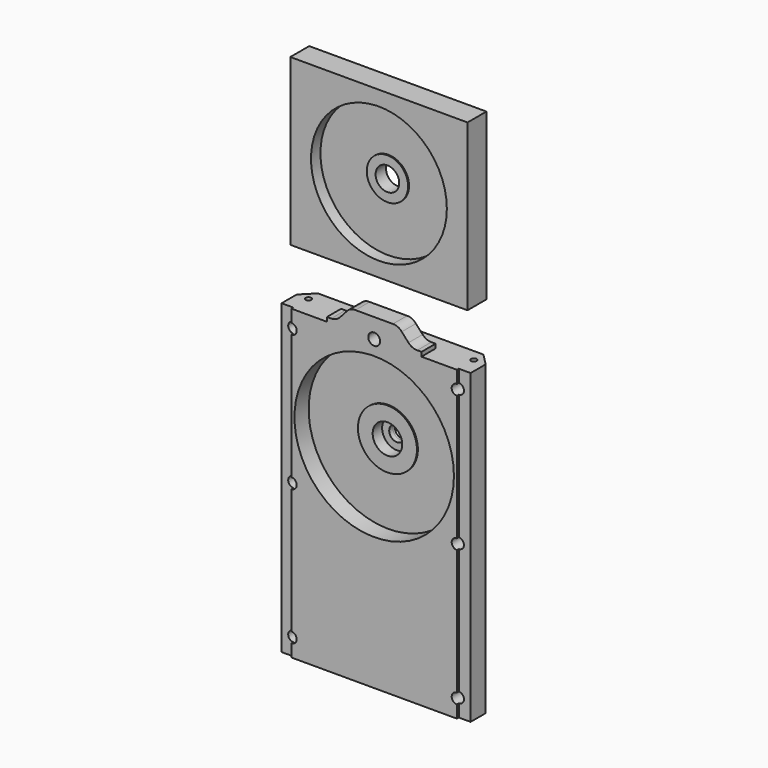
from build123d import *
from build123d import SkipClean  # not in build123d's __all__

# Parameters (mm, degrees)
F0_R            = 3.25
F1_DEPTH        = 6.5
F2_R            = 33.75
F3_DEPTH        = 7.5
F4_R            = 12.5
F4_R_2          = 3.25
F5_DEPTH        = 0.5
F6_R            = 8.25
F6_R_2          = 3.25
F7_DEPTH        = 1
F9_DEPTH        = 50
F10_DEPTH       = 120
F12_D           = 4.4
F12_CBORE_D     = 8.25
F12_CBORE_DEPTH = 4
F13_T1_DEPTH    = 155.7168298797
F14_R           = 2.5
F15_DEPTH       = 15.001
F16_R           = 4.8
F17_DEPTH       = 5
F18_R           = 3.3
F19_DEPTH       = 2.5
F20_R           = 4.8
F21_DEPTH       = 0.1
F23_DEPTH       = 1
F24_R           = 6.25
F25_DEPTH       = 5
F27_D           = 2.4
F27_DEPTH       = 2.5
F27_TIP         = 0.7210327428
F28_W           = 75
F28_H           = 70
F28_R           = 5
F29_DEPTH       = 5
F30_W           = 75
F30_H           = 70
F30_R           = 28.75
F31_DEPTH       = 5
F32_R           = 8.75
F32_R_2         = 5
F33_DEPTH       = 0.5


# Not quite as in the source:
# - a fillet or chamfer that OpenCascade refuses, or shapes differently, is made with other operations: its cross-section is extruded or revolved along the edge and cut away or added
# - after a boolean that leaves OpenCascade's solid faulty, fix() repairs it
# - a feature names something its author has since deleted; it is built from what else it names


with BuildPart() as f1:
    # F0 (on Front) → F1 (new body)
    with BuildSketch(Plane.XZ):
        Polygon((40, -40), (40, -23.2305045641), (40, 0.7694954359), (40, 40), (19.3889045436, 40), (-20.6110954564, 40), (-40, 40), (-40, 0.7694954359), (-40, -23.2305045641), (-40, -40), align=None)
        Circle(F0_R, mode=Mode.SUBTRACT)
    extrude(amount=-F1_DEPTH)

    # F2 (on Front) → F3 (join)
    with BuildSketch(Plane.XZ):
        with BuildLine():
            Line((-40, 40), (-40, -40))
            Line((-40, -40), (40, -40))
            Line((40, -40), (40, 40))
            Line((40, 40), (20, 40))
            Line((20, 40), (20, 41.789))
            Line((20, 41.789), (18.202, 41.789))
            ThreePointArc((18.202, 41.789), (16.1810670348, 42.2156172312), (14.505, 43.4226680199))
            Line((14.505, 43.4226680199), (11.656, 46.56))
            ThreePointArc((11.656, 46.56), (9.9989699318, 47.8636778232), (7.93, 48.2694954359))
            Line((7.93, 48.2694954359), (-7.93, 48.2694954359))
            ThreePointArc((-7.93, 48.2694954359), (-9.9989699318, 47.8636778232), (-11.656, 46.56))
            Line((-11.656, 46.56), (-14.505, 43.4226680199))
            ThreePointArc((-14.505, 43.4226680199), (-16.1810670348, 42.2156172312), (-18.202, 41.789))
            Line((-18.202, 41.789), (-20, 41.789))
            Line((-20, 41.789), (-20, 40))
            Line((-20, 40), (-40, 40))
        make_face()
        Circle(F2_R, mode=Mode.SUBTRACT)
    extrude(amount=F3_DEPTH)

    # F4 (on face) → F5 (join)
    with BuildSketch(Plane.XZ):
        Circle(F4_R)
        Circle(F4_R_2, mode=Mode.SUBTRACT)
    extrude(amount=F5_DEPTH)

    # F6 (on face) → F7 (join)
    with BuildSketch(Plane(origin=(0, 6.5, 0), x_dir=(-1, 0, 0), z_dir=(0, 1, 0))):
        Circle(F6_R)
        Circle(F6_R_2, mode=Mode.SUBTRACT)
    with SkipClean():  # cleaning this boolean's faces spoils the solid; the shape is the same uncleaned
        extrude(amount=F7_DEPTH)

    # F8 (on face) → F9 (join)
    with BuildSketch(Plane(origin=(0, 0, -40), x_dir=(1, 0, 0), z_dir=(0, 0, -1))):
        Polygon((27.5, -6.5), (40, -6.5), (40, 6.5), (35, 6.5), (35, 7.5), (-35, 7.5), (-35, 6.5), (-40, 6.5), (-40, -6.5), (-27.5, -6.5), (-27.5, 2.5), (27.5, 2.5), align=None)
    extrude(amount=F9_DEPTH)

    add(f1.part.fix(), mode=Mode.REPLACE)

    # F10 (cut): faces of the model
    f10_faces = [f1.faces().sort_by_distance(p)[0] for p in [
        (37.5, -7, -40),
        (-37.5, -7, -40),
    ]]
    extrude(f10_faces, amount=-F10_DEPTH, mode=Mode.SUBTRACT)

    # F12 (through all)
    with Locations(Plane(origin=(0, 6.5, 0), x_dir=(-1, 0, 0), z_dir=(0, 1, 0))):
        with Locations((35, 32.5), (35, -25), (35, -82.5), (-35, -82.5), (-35, -25), (-35, 32.5)):
            CounterBoreHole(F12_D / 2, F12_CBORE_D / 2, F12_CBORE_DEPTH)

    # F13: chamfer of 5 on 2 edges, made by hand

    # F13_s2 → F13_t1 (cut)
    with BuildSketch(Plane.XY.offset(-102.8584149398)):
        Polygon((40, 1.5), (35, 6.5), (40, 6.5), align=None)
        Polygon((-35, 6.5), (-40, 1.5), (-40, 6.5), align=None)
    extrude(amount=F13_T1_DEPTH, mode=Mode.SUBTRACT)

    # F14 (on face) → F15 (cut, through all)
    with BuildSketch(Plane.XZ.offset(7.5)):
        with Locations((0, 40)):
            Circle(F14_R)
    extrude(amount=-F15_DEPTH, mode=Mode.SUBTRACT)

    # F16 (on Front) → F17 (cut)
    with BuildSketch(Plane.XZ):
        with Locations((0, 40)):
            Circle(F16_R)
    extrude(amount=-F17_DEPTH, mode=Mode.SUBTRACT)

    # F18 (on face) → F19 (cut)
    with BuildSketch(Plane(origin=(0, 6.5, 0), x_dir=(-1, 0, 0), z_dir=(0, 1, 0))):
        with Locations((0, 40)):
            Circle(F18_R)
    extrude(amount=-F19_DEPTH, mode=Mode.SUBTRACT)

    # F20 (on face) → F21 (cut)
    with BuildSketch(Plane(origin=(0, 0, 0), x_dir=(-1, 0, 0), z_dir=(0, 1, 0))):
        with Locations((0, 40)):
            Circle(F20_R)
    extrude(amount=-F21_DEPTH, mode=Mode.SUBTRACT)

    # F22 (on face) → F23 (join)
    with BuildSketch(Plane(origin=(0, 6.5, 0), x_dir=(-1, 0, 0), z_dir=(0, 1, 0))):
        with BuildLine():
            ThreePointArc((3.3, 40), (0, 36.7), (-3.3, 40))
            Line((-3.3, 40), (-6.25, 40))
            ThreePointArc((-6.25, 40), (0, 33.75), (6.25, 40))
            Line((6.25, 40), (3.3, 40))
        make_face()
    extrude(amount=F23_DEPTH)

    # F24 (on face) → F25 (cut)
    with BuildSketch(Plane.XZ.offset(0.5)):
        Circle(F24_R)
    extrude(amount=-F25_DEPTH, mode=Mode.SUBTRACT)

    # F27
    with Locations(Plane.XY.offset(40)):
        with Locations((-35, 1.5), (35, 1.5)):
            Hole(F27_D / 2, depth=F27_DEPTH)
            with Locations((0, 0, -(F27_DEPTH + F27_TIP / 2))):  # 118° drill point
                Cone(0, F27_D / 2, F27_TIP, mode=Mode.SUBTRACT)


with BuildPart() as f29:
    # F28 (on Front) → F29 (new body)
    with BuildSketch(Plane.XZ):
        with Locations((0, 96.9531931057)):
            Rectangle(F28_W, F28_H)
        with Locations((0, 96.9531931057)):
            Circle(F28_R, mode=Mode.SUBTRACT)
    extrude(amount=-F29_DEPTH)

    # F30 (on face) → F31 (join)
    with BuildSketch(Plane.XZ):
        with Locations((0, 96.9531931057)):
            Rectangle(F30_W, F30_H)
        with Locations((0, 96.9531931057)):
            Circle(F30_R, mode=Mode.SUBTRACT)
    extrude(amount=F31_DEPTH)

    # F32 (on face) → F33 (join)
    with BuildSketch(Plane.XZ):
        with Locations((0, 96.9531931057)):
            Circle(F32_R)
        with Locations((0, 96.9531931057)):
            Circle(F32_R_2, mode=Mode.SUBTRACT)
    extrude(amount=F33_DEPTH)


solid = Compound([f1.part, f29.part])
